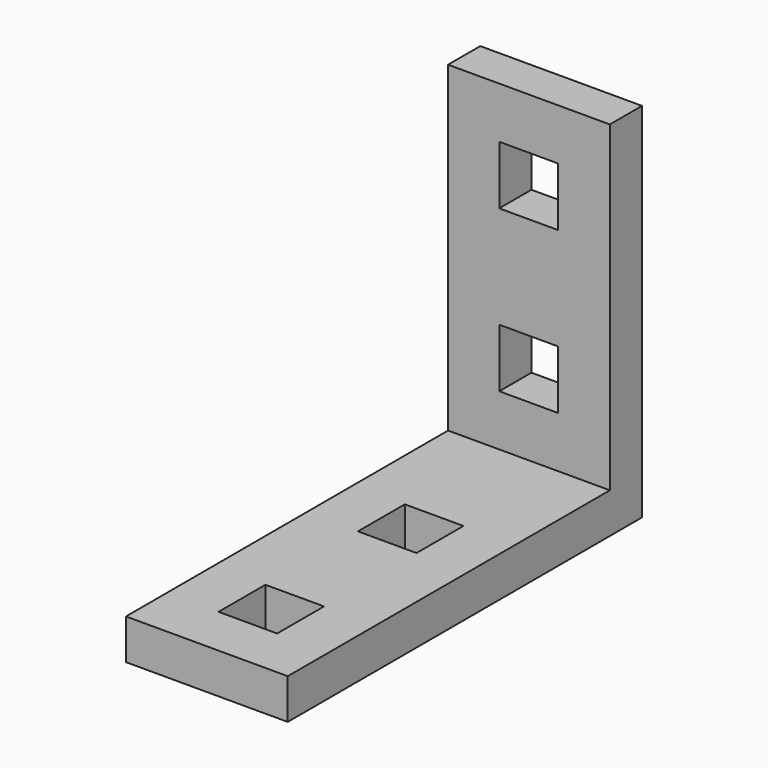
from build123d import *

# Parameters (mm, degrees)
F0_W     = 4.6228
F0_H     = 4.6228
F1_DEPTH = 3.175
F2_DEPTH = 34.925
F3_W     = 4.6228
F3_H     = 4.6228
F4_DEPTH = 25.4


with BuildPart() as f1:
    # F0 (on Front) → F1 (new body)
    with BuildSketch(Plane.XZ):
        Polygon((6.37921, -9.525), (6.37921, 15.875), (-6.37921, 15.875), (-6.37921, -9.525), (-1.8334548599, -9.525), align=None)
        with Locations((-0.02921, -3.175)):
            Rectangle(F0_W, F0_H, mode=Mode.SUBTRACT)
        with Locations((-0.02921, 9.525)):
            Rectangle(F0_W, F0_H, mode=Mode.SUBTRACT)
    extrude(amount=F1_DEPTH)

    # F0 (on Front) → F2 (join)
    with BuildSketch(Plane.XZ):
        Polygon((6.37921, -12.7), (6.37921, -9.525), (-1.8334548599, -9.525), (-6.37921, -9.525), (-6.37921, -12.7), (2.7123002801, -12.7), align=None)
    extrude(amount=F2_DEPTH)

    # F3 (on face) → F4 (cut)
    with BuildSketch(Plane.XY.offset(-9.525)):
        with Locations((0, -14.8336)):
            Rectangle(F3_W, F3_H)
        Polygon((-2.3114, -30.8864), (0, -30.8864), (2.3114, -30.8864), (2.3114, -26.2636), (-2.3114, -26.2636), align=None)
    extrude(amount=-F4_DEPTH, mode=Mode.SUBTRACT)


solid = f1.part
